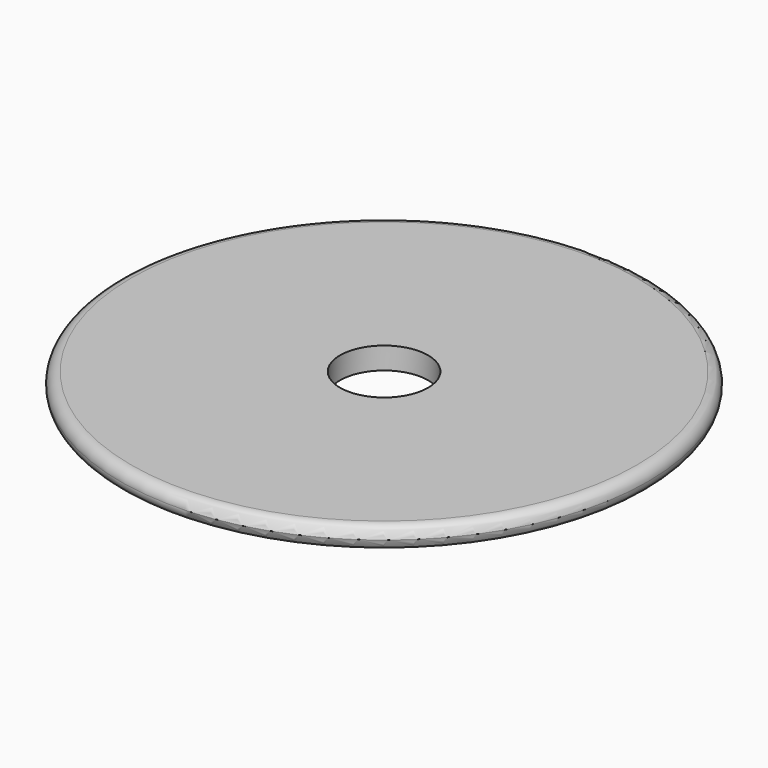
from build123d import *

# Parameters (mm, degrees)
F0_R     = 19.05
F0_R_2   = 3.175
F1_DEPTH = 1.5875
F2_R     = 0.79374


# Not quite as in the source:
# - a fillet or chamfer is up to 0.001 mm smaller than in the source, because OpenCascade refuses the exact size


with BuildPart() as f1:
    # F0 (on Top) → F1 (new body)
    with BuildSketch(Plane.XY):
        Circle(F0_R)
        Circle(F0_R_2, mode=Mode.SUBTRACT)
    extrude(amount=F1_DEPTH)

    # F2 (radius 0.79375 in the source; OpenCascade refuses exactly that, so slightly less here)
    f2_edges = [f1.edges().sort_by_distance(p)[0] for p in [
        (19.05, 0, 0.79375),
        (-19.05, 0, 0),
        (-19.05, 0, 1.5875),
    ]]
    fillet(f2_edges, radius=F2_R)


solid = f1.part
